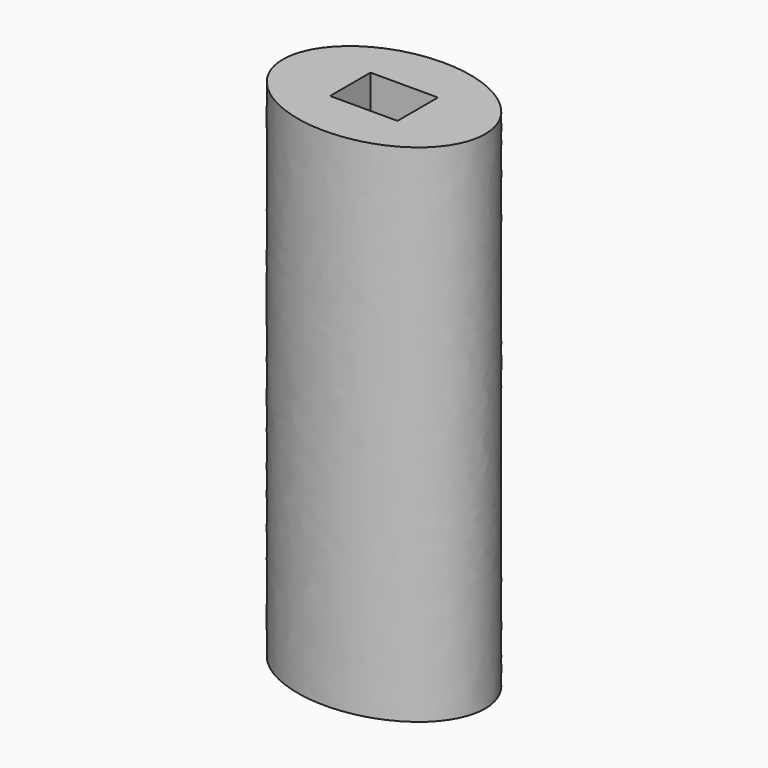
from build123d import *

# Parameters (mm, degrees)
F1_DEPTH = 150
F3_W     = 20
F3_H     = 15
F4_DEPTH = 70


# Not quite as in the source:
# - a feature names something its author has since deleted; it is built from what else it names


with BuildPart() as f1:
    # F0 (on Top) → F1 (new body)
    with BuildSketch(Plane.XY):
        with BuildLine():
            add(Edge.make_bspline(
                [(-30, 0), (-30, -38.1051177665), (15, -19.0525588833), (60, 0), (15, 19.0525588833), (-30, 38.1051177665), (-30, 0)],
                knots=[0, 0, 0, 2.0943951024, 2.0943951024, 4.1887902048, 4.1887902048, 6.2831853072, 6.2831853072, 6.2831853072], degree=2, weights=[1, 0.5, 1, 0.5, 1, 0.5, 1]))
        make_face()
    extrude(amount=F1_DEPTH)

    # F3 (on face) → F4 (cut)
    with BuildSketch(Plane.XY.offset(150)):
        Rectangle(F3_W, F3_H)
    extrude(amount=-F4_DEPTH, mode=Mode.SUBTRACT)


solid = f1.part
